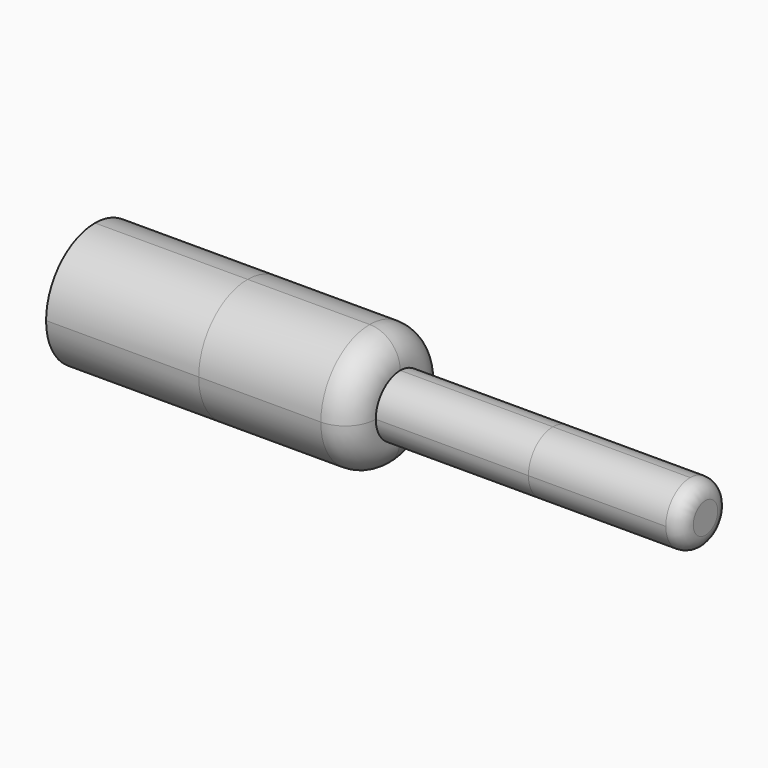
from build123d import *

# Parameters (mm, degrees)
F1_DEPTH = 254
F2_DEPTH = 190.5
F3_DEPTH = 127
F4_DEPTH = 63.5
F5_R     = 12.6999
F6_R     = 25.3999
F7_R     = 12.6999


# Not quite as in the source:
# - a fillet or chamfer that OpenCascade refuses, or shapes differently, is made with other operations: its cross-section is extruded or revolved along the edge and cut away or added
# - a fillet or chamfer is up to 0.001 mm smaller than in the source, because OpenCascade refuses the exact size


with BuildPart() as f1:
    # F0 (on Right) → F1 (new body)
    with BuildSketch(Plane.YZ):
        with BuildLine():
            ThreePointArc((12.7, 0), (8.9802561211, 8.9802561211), (0, 12.7))
            ThreePointArc((0, 12.7), (-8.9802561211, 8.9802561211), (-12.7, 0))
            ThreePointArc((-12.7, 0), (-8.9802561211, -8.9802561211), (0, -12.7))
            ThreePointArc((0, -12.7), (8.9802561211, -8.9802561211), (12.7, 0))
        make_face()
    extrude(amount=F1_DEPTH)

    # F0 (on Right) → F2 (join)
    with BuildSketch(Plane.YZ):
        with BuildLine():
            ThreePointArc((-12.7, 0), (-8.9802561211, 8.9802561211), (0, 12.7))
            Line((0, 12.7), (-12.7, 12.7))
            Line((-12.7, 12.7), (-12.7, 0))
        make_face()
        with BuildLine():
            Line((12.7, 12.7), (0, 12.7))
            ThreePointArc((0, 12.7), (8.9802561211, 8.9802561211), (12.7, 0))
            Line((12.7, 0), (12.7, 12.7))
        make_face()
        with BuildLine():
            Line((12.7, -12.7), (12.7, 0))
            ThreePointArc((12.7, 0), (8.9802561211, -8.9802561211), (0, -12.7))
            Line((0, -12.7), (12.7, -12.7))
        make_face()
        with BuildLine():
            ThreePointArc((0, -12.7), (-8.9802561211, -8.9802561211), (-12.7, 0))
            Line((-12.7, 0), (-12.7, -12.7))
            Line((-12.7, -12.7), (0, -12.7))
        make_face()
    extrude(amount=F2_DEPTH)

    # F0 (on Right) → F3 (join)
    with BuildSketch(Plane.YZ):
        with BuildLine():
            ThreePointArc((25.4, 0), (17.9605122421, 17.9605122421), (0, 25.4))
            ThreePointArc((0, 25.4), (-17.9605122421, 17.9605122421), (-25.4, 0))
            ThreePointArc((-25.4, 0), (-17.9605122421, -17.9605122421), (0, -25.4))
            ThreePointArc((0, -25.4), (17.9605122421, -17.9605122421), (25.4, 0))
        make_face()
        Polygon((-12.7, 12.7), (0, 12.7), (12.7, 12.7), (12.7, 0), (12.7, -12.7), (0, -12.7), (-12.7, -12.7), (-12.7, 0), align=None, mode=Mode.SUBTRACT)
    extrude(amount=F3_DEPTH)

    # F0 (on Right) → F4 (join)
    with BuildSketch(Plane.YZ):
        with BuildLine():
            ThreePointArc((-25.4, 0), (-17.9605122421, 17.9605122421), (0, 25.4))
            Line((0, 25.4), (-25.4, 25.4))
            Line((-25.4, 25.4), (-25.4, 0))
        make_face()
        with BuildLine():
            ThreePointArc((0, -25.4), (-17.9605122421, -17.9605122421), (-25.4, 0))
            Line((-25.4, 0), (-25.4, -25.4))
            Line((-25.4, -25.4), (0, -25.4))
        make_face()
        with BuildLine():
            Line((25.4, -25.4), (25.4, 0))
            ThreePointArc((25.4, 0), (17.9605122421, -17.9605122421), (0, -25.4))
            Line((0, -25.4), (25.4, -25.4))
        make_face()
        with BuildLine():
            Line((25.4, 25.4), (0, 25.4))
            ThreePointArc((0, 25.4), (17.9605122421, 17.9605122421), (25.4, 0))
            Line((25.4, 0), (25.4, 25.4))
        make_face()
    extrude(amount=F4_DEPTH)

    # F5 (radius 12.7 in the source; OpenCascade refuses exactly that, so slightly less here)
    f5_edges = [f1.edges().sort_by_distance(p)[0] for p in [
        (158.75, -12.7, -12.7),
        (158.75, 12.7, -12.7),
        (158.75, 12.7, 12.7),
        (158.75, -12.7, 12.7),
    ]]
    fillet(f5_edges, radius=F5_R)

    # F6 (radius 25.4 in the source; OpenCascade refuses exactly that, so slightly less here)
    f6_edges = [f1.edges().sort_by_distance(p)[0] for p in [
        (31.75, -25.4, -25.4),
        (31.75, 25.4, -25.4),
        (31.75, -25.4, 25.4),
        (31.75, 25.4, 25.4),
    ]]
    fillet(f6_edges, radius=F6_R)

    # F7 (radius 12.7 in the source; OpenCascade refuses exactly that, so slightly less here)
    f7_edges = [f1.edges().sort_by_distance(p)[0] for p in [
        (127, 25.4, 0),
    ]]
    fillet(f7_edges, radius=F7_R)

    # F8: fillet of radius 6.35 on 1 edges, made by hand

    # F8_s1 → F8_t2 (revolve, cut)
    with BuildSketch(Plane.XY):
        with BuildLine():
            ThreePointArc((247.65, -12.7), (252.1401280605, -10.8401280605), (254, -6.35))
            Line((254, -6.35), (254, -12.7))
            Line((254, -12.7), (247.65, -12.7))
        make_face()
    revolve(axis=Axis((254, 0, 0), (-1, 0, 0)), mode=Mode.SUBTRACT)


solid = f1.part
